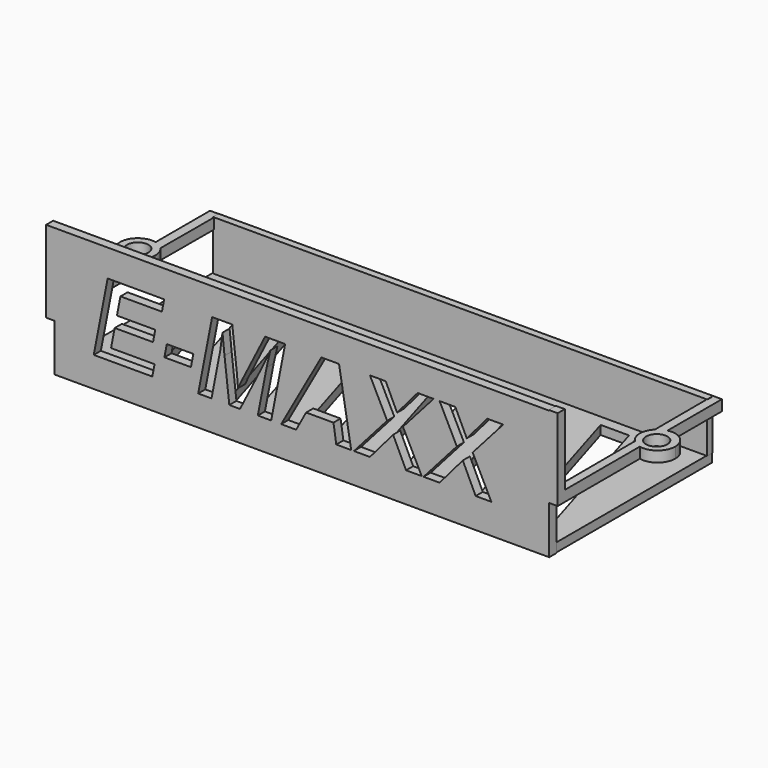
from build123d import *

# Parameters (mm, degrees)
F0_W     = 139
F0_H     = 55
F1_DEPTH = 2.5
F2_W     = 2.3327280719
F2_H     = 23
F2_W_2   = 0.1672719281
F2_W_3   = 0.1289593171
F2_H_2   = 22.8627715209
F3_DEPTH = 2.5
F5_DEPTH = 3
F6_W     = 139
F6_H     = 1.9677817641
F7_DEPTH = 14
F9_D     = 6


with BuildPart() as f1:
    # F0 (on Top) → F1 (new body)
    with BuildSketch(Plane.XY):
        with Locations((3.418983344, 2.2497611304)):
            Rectangle(F0_W, F0_H)
        Polygon((-46.7749163508, -16.9449970126), (-59.4031140208, 24.8976889998), (-51.4031140208, 24.8976889998), (-38.7749163508, -16.9449970126), align=None, mode=Mode.SUBTRACT)
        Polygon((-25.7749595437, -16.9785083988), (-38.4031572137, 24.8641776135), (-30.4031572137, 24.8641776135), (-17.7749595437, -16.9785083988), align=None, mode=Mode.SUBTRACT)
        Polygon((-4.7749595437, -17.1519126743), (-17.4031572137, 24.6907733381), (-9.4031572137, 24.6907733381), (3.2250404563, -17.1519126743), align=None, mode=Mode.SUBTRACT)
        Polygon((16.2250404563, -17.1519108117), (3.5968427863, 24.6907752007), (11.5968427863, 24.6907752007), (24.2250404563, -17.1519108117), align=None, mode=Mode.SUBTRACT)
        Polygon((37.2244375112, -17.277115479), (24.5962398412, 24.5655705334), (32.5962398412, 24.5655705334), (45.2244375112, -17.277115479), align=None, mode=Mode.SUBTRACT)
        Polygon((58.2235167211, -17.1223909005), (45.5953190511, 24.7202951119), (53.5953190511, 24.7202951119), (66.2235167211, -17.1223909005), align=None, mode=Mode.SUBTRACT)
    extrude(amount=F1_DEPTH)

    # F2 (on face) → F3 (join)
    with BuildSketch(Plane.XZ.offset(25.2502388696)):
        Polygon((-66.081016656, 13.302537529), (-66.081016656, 0), (73.1178743134, 0), (73.1178743134, 13.4397660082), (72.9889149964, 13.4397660082), (72.9889149964, 36.302537529), (-65.9137447279, 36.302537529), (-65.9137447279, 13.302537529), align=None)
        Polygon((-27.6715531448, 14.3061928175), (-35.129489078, 14.3061928175), (-34.4548327198, 17.8079805818), (-26.9968967865, 17.8079805818), align=None, mode=Mode.SUBTRACT)
        Polygon((-38.5440763607, 8.4408130497), (-55.0066094022, 8.4408130497), (-51.0917667246, 28.6483773044), (-35.2029210626, 28.6483773044), (-35.8316824305, 25.3806539909), (-47.4935994805, 25.3806539909), (-48.4849312723, 20.3000785582), (-37.6996085381, 20.3000785582), (-38.328369906, 17.0323552447), (-49.1136926402, 17.0323552447), (-50.1463299232, 11.7131258622), (-37.8969569966, 11.7131258622), align=None, mode=Mode.SUBTRACT)
        with BuildLine():
            Line((-5.0958073876, 8.4408130497), (-8.8546070979, 8.4408130497))
            Line((-8.8546070979, 8.4408130497), (-6.3900461157, 21.1215988857))
            add(Edge.make_bspline(
                [(-6.3900461157, 21.1215988857), (-6.0137071947, 22.9849354942), (-5.3252823394, 25.7386349157)],
                knots=[0, 0, 0, 1, 1, 1], degree=2))
            Line((-5.3252823394, 25.7386349157), (-6.3166141311, 23.5723913708))
            add(Edge.make_bspline(
                [(-6.3166141311, 23.5723913708), (-7.450220393, 21.0757038953), (-7.9504757879, 20.144035591)],
                knots=[0, 0, 0, 1, 1, 1], degree=2))
            Line((-7.9504757879, 20.144035591), (-13.861750546, 8.4408130497))
            Line((-13.861750546, 8.4408130497), (-16.8724619135, 8.4408130497))
            Line((-16.8724619135, 8.4408130497), (-18.22177463, 20.1853410823))
            add(Edge.make_bspline(
                [(-18.22177463, 20.1853410823), (-18.6669560365, 24.3617852049), (-18.7954620095, 25.7386349157)],
                knots=[0, 0, 0, 1, 1, 1], degree=2))
            add(Edge.make_bspline(
                [(-18.7954620095, 25.7386349157), (-19.1947484256, 22.2368471514), (-19.4104548803, 21.162904377)],
                knots=[0, 0, 0, 1, 1, 1], degree=2))
            Line((-19.4104548803, 21.162904377), (-21.8796053616, 8.4408130497))
            Line((-21.8796053616, 8.4408130497), (-25.6338155729, 8.4408130497))
            Line((-25.6338155729, 8.4408130497), (-21.7052043982, 28.6483773044))
            Line((-21.7052043982, 28.6483773044), (-16.041762588, 28.6483773044))
            Line((-16.041762588, 28.6483773044), (-14.7796503532, 17.3490306782))
            Line((-14.7796503532, 17.3490306782), (-14.4216694284, 13.3882930103))
            add(Edge.make_bspline(
                [(-14.4216694284, 13.3882930103), (-13.9030560373, 14.5356677692), (-13.4578746309, 15.4673360735)],
                knots=[0, 0, 0, 1, 1, 1], degree=2))
            add(Edge.make_bspline(
                [(-13.4578746309, 15.4673360735), (-13.0126932244, 16.3990043778), (-6.8031010289, 28.6483773044)],
                knots=[0, 0, 0, 1, 1, 1], degree=2))
            Line((-6.8031010289, 28.6483773044), (-1.1671962129, 28.6483773044))
            Line((-1.1671962129, 28.6483773044), (-5.0958073876, 8.4408130497))
        make_face(mode=Mode.SUBTRACT)
        Polygon((17.401916886, 8.4408130497), (13.2162937654, 8.4408130497), (12.4268999312, 13.603999465), (4.7257205491, 13.603999465), (1.9307156363, 8.4408130497), (-2.2870339777, 8.4408130497), (8.9985441514, 28.6483773044), (13.9919191024, 28.6483773044), align=None, mode=Mode.SUBTRACT)
        Polygon((27.5309412581, 18.9966608321), (22.6844302763, 28.6483773044), (27.1132968458, 28.6483773044), (30.3259461709, 21.8926347237), (36.0903569599, 28.6483773044), (40.583476516, 28.6483773044), (31.9781658238, 18.9415868436), (37.2377317189, 8.4408130497), (32.8364021435, 8.4408130497), (29.2061084062, 16.0731499462), (22.6844302763, 8.4408130497), (18.1775422231, 8.4408130497), align=None, mode=Mode.SUBTRACT)
        Polygon((47.123512642, 18.9966608321), (42.2770016602, 28.6483773044), (46.7058682298, 28.6483773044), (49.9185175548, 21.8926347237), (55.6829283438, 28.6483773044), (60.1760478999, 28.6483773044), (51.5707372077, 18.9415868436), (56.8303031028, 8.4408130497), (52.4289735274, 8.4408130497), (48.7986797901, 16.0731499462), (42.2770016602, 8.4408130497), (37.770113607, 8.4408130497), align=None, mode=Mode.SUBTRACT)
        with Locations((-67.247380692, 24.802537529)):
            Rectangle(F2_W, F2_H)
        with Locations((-65.997380692, 24.802537529)):
            Rectangle(F2_W_2, F2_H)
        with Locations((73.0533946549, 24.8711517686)):
            Rectangle(F2_W_3, F2_H_2)
        Polygon((73.1178743134, 36.302537529), (73.1178743134, 13.4397660082), (75.4889149964, 13.4397660082), (75.4889149964, 36.4397660082), (72.9889149964, 36.4397660082), (72.9889149964, 36.302537529), align=None)
    extrude(amount=F3_DEPTH)

    # F4 (on face) → F5 (join)
    with BuildSketch(Plane(origin=(0, 0, 13.4397660082), x_dir=(1, 0, 0), z_dir=(0, 0, -1))):
        with BuildLine():
            Line((75.4889149964, 25.2502388696), (75.4889149964, 27.7502388696))
            Line((75.4889149964, 27.7502388696), (73.1178743134, 27.7502388696))
            Line((73.1178743134, 27.7502388696), (73.1178743134, 25.2502388696))
            Line((73.1178743134, 25.2502388696), (73.0357726252, -2.464520624))
            ThreePointArc((73.0357726252, -2.464520624), (74.1664237205, -1.6173558789), (75.4889149964, -1.1202876444))
            Line((75.4889149964, -1.1202876444), (75.4889149964, 25.2502388696))
        make_face()
        with BuildLine():
            ThreePointArc((81.5691593623, -6.0022003956), (79.6995569545, -2.1034043102), (75.4889149964, -1.1202876444))
            Line((75.4889149964, -1.1202876444), (75.4889149964, -10.8841131467))
            ThreePointArc((75.4889149964, -10.8841131467), (79.6995569545, -9.9009964809), (81.5691593623, -6.0022003956))
        make_face()
        with BuildLine():
            Line((75.4889149964, -10.8841131467), (75.4889149964, -1.1202876444))
            ThreePointArc((75.4889149964, -1.1202876444), (74.1664237205, -1.6173558789), (73.0357726252, -2.464520624))
            Line((73.0357726252, -2.464520624), (73.014874911, -9.5188837818))
            ThreePointArc((73.014874911, -9.5188837818), (74.1534447384, -10.3799078842), (75.4889149964, -10.8841131467))
        make_face()
        with BuildLine():
            Line((75.4889149964, -30.0022003956), (75.4889149964, -10.8841131467))
            ThreePointArc((75.4889149964, -10.8841131467), (74.1534447384, -10.3799078842), (73.014874911, -9.5188837818))
            Line((73.014874911, -9.5188837818), (72.9604437947, -27.8929919004))
            Line((72.9604437947, -27.8929919004), (61.0808953643, -27.8929919004))
            Line((61.0808953643, -27.8929919004), (61.0808953643, -30.0022003956))
            Line((61.0808953643, -30.0022003956), (75.4889149964, -30.0022003956))
        make_face()
        with BuildLine():
            Line((73.014874911, -9.5188837818), (73.0357726252, -2.464520624))
            ThreePointArc((73.0357726252, -2.464520624), (71.5691813014, -5.9873885535), (73.014874911, -9.5188837818))
        make_face()
        with BuildLine():
            Line((-68.1669373373, 27.6543483512), (-68.3165375451, 27.5479025488))
            Line((-68.3165375451, 27.5479025488), (-68.3165375451, -0.8886232584))
            ThreePointArc((-68.3165375451, -0.8886232584), (-66.8972077442, -1.452270315), (-65.714216699, -2.4180483823))
            Line((-65.714216699, -2.4180483823), (-65.7958966544, 25.1543483512))
            Line((-65.7958966544, 25.1543483512), (-65.7958966544, 27.6543483512))
            Line((-65.7958966544, 27.6543483512), (-68.1669373373, 27.6543483512))
        make_face()
        with BuildLine():
            ThreePointArc((-65.714216699, -2.4180483823), (-66.8972077442, -1.452270315), (-68.3165375451, -0.8886232584))
            Line((-68.3165375451, -0.8886232584), (-68.3165375451, -10.637216093))
            ThreePointArc((-68.3165375451, -10.637216093), (-66.884449129, -10.0660451489), (-65.6944645318, -9.0857135021))
            Line((-65.6944645318, -9.0857135021), (-65.714216699, -2.4180483823))
        make_face()
        with BuildLine():
            Line((-68.3165375451, -10.637216093), (-68.3165375451, -0.8886232584))
            ThreePointArc((-68.3165375451, -0.8886232584), (-74.4306445579, -5.7629196757), (-68.3165375451, -10.637216093))
        make_face()
        with BuildLine():
            ThreePointArc((-65.6944645318, -9.0857135021), (-66.884449129, -10.0660451489), (-68.3165375451, -10.637216093))
            Line((-68.3165375451, -10.637216093), (-68.3165375451, -29.7629196757))
            Line((-68.3165375451, -29.7629196757), (-53.7589177052, -29.8940964603))
            Line((-53.7589177052, -29.8940964603), (-53.7589177052, -27.9888824189))
            Line((-53.7589177052, -27.9888824189), (-61.1505493085, -27.9888824189))
            Line((-61.1505493085, -27.9888824189), (-65.6384661357, -27.9888824189))
            Line((-65.6384661357, -27.9888824189), (-65.6944645318, -9.0857135021))
        make_face()
        with BuildLine():
            ThreePointArc((-64.4306445579, -5.7629196757), (-64.7625539796, -3.9715709233), (-65.714216699, -2.4180483823))
            Line((-65.714216699, -2.4180483823), (-65.6944645318, -9.0857135021))
            ThreePointArc((-65.6944645318, -9.0857135021), (-64.7572678274, -7.5404319639), (-64.4306445579, -5.7629196757))
        make_face()
    extrude(amount=-F5_DEPTH)

    # F6 (on face) → F7 (join)
    with BuildSketch(Plane.XY.offset(2.5)):
        with Locations((3.5998241897, 28.7658702483)):
            Rectangle(F6_W, F6_H)
    extrude(amount=F7_DEPTH)

    # F9 (through all)
    with Locations(Plane.XY.offset(16.4397660082)):
        with Locations((-69.4306445579, 5.7629196757), (76.5447840095, 5.7629196757)):
            Hole(F9_D / 2)


solid = f1.part
